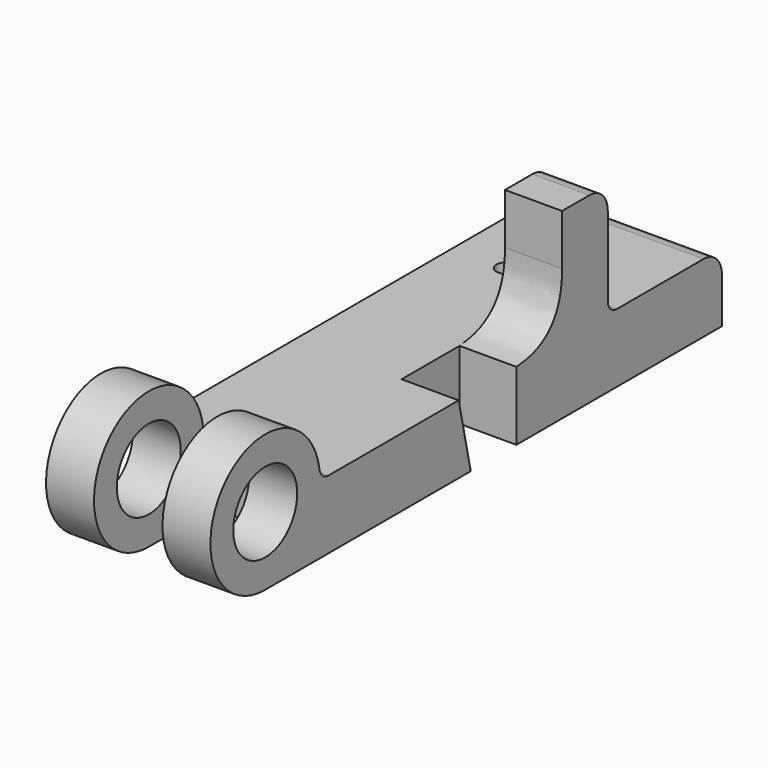
from build123d import *

# Parameters (mm, degrees)
F0_R         = 7
F1_DEPTH     = 14.4
F2_W         = 12
F2_H         = 26.4532811218
F2_H_2       = 2.4532811218
F3_DEPTH     = 15
F4_R         = 2
F6_DEPTH     = 25
F7_W         = 18.8
F7_H         = 33.2335345083
F7_H_2       = 13.5664814711
F8_DEPTH     = 25
F11_DEPTH    = 10
F12_T4_DEPTH = 10


# Not quite as in the source:
# - a fillet or chamfer that OpenCascade refuses, or shapes differently, is made with other operations: its cross-section is extruded or revolved along the edge and cut away or added


with BuildPart() as f1:
    # F0 (on Right) → F1 (new body, symmetric)
    with BuildSketch(Plane.YZ):
        with BuildLine():
            Line((42.36, 0), (12, 0))
            ThreePointArc((12, 0), (-8.4852813742, 8.4852813742), (0, -12))
            Line((0, -12), (47.36, -12))
            Line((47.36, -12), (42.36, 0))
        make_face()
        Circle(F0_R, mode=Mode.SUBTRACT)
        Polygon((57.36, 0), (42.36, 0), (47.36, -12), (57.36, -12), align=None)
        with BuildLine():
            Line((65, 0), (57.36, 0))
            Line((57.36, 0), (57.36, -12))
            Line((57.36, -12), (100, -12))
            Line((100, -12), (100, -4))
            ThreePointArc((100, -4), (98.8284271247, -1.1715728753), (96, 0))
            Line((96, 0), (77, 0))
            ThreePointArc((77, 0), (75.5857864376, 0.5857864376), (75, 2))
            Line((75, 2), (75, 16))
            ThreePointArc((75, 16), (73.8284271247, 18.8284271247), (71, 20))
            Line((71, 20), (65, 20))
            Line((65, 20), (65, 0))
        make_face()
    extrude(amount=F1_DEPTH, both=True)

    # F2 (on face) → F3 (cut, symmetric)
    with BuildSketch(Plane.XY):
        with Locations((0, -1.2266405609)):
            Rectangle(F2_W, F2_H)
        with Locations((0, 13.2266405609)):
            Rectangle(F2_W, F2_H_2)
    extrude(amount=F3_DEPTH, both=True, mode=Mode.SUBTRACT)

    # F4
    f4_edges = [f1.edges().sort_by_distance(p)[0] for p in [
        (10.2, 12, 0),
        (-10.2, 12, 0),
    ]]
    fillet(f4_edges, radius=F4_R)

    # F5 (on face) → F6 (cut)
    with BuildSketch(Plane.XY):
        with BuildLine():
            Line((-5, 77), (-6.7, 77))
            ThreePointArc((-6.7, 77), (-5, 75.3), (-3.3, 77))
            Line((-3.3, 77), (-5, 77))
        make_face()
        with BuildLine():
            ThreePointArc((-3.3, 77), (-5, 78.7), (-6.7, 77))
            Line((-6.7, 77), (-5, 77))
            Line((-5, 77), (-3.3, 77))
        make_face()
    extrude(amount=-F6_DEPTH, mode=Mode.SUBTRACT)

    # F7 (on face) → F8 (cut)
    with BuildSketch(Plane.XY):
        with Locations((-5, 81.6167672542)):
            Rectangle(F7_W, F7_H)
        with Locations((-5, 58.2167592645)):
            Rectangle(F7_W, F7_H_2)
    extrude(amount=F8_DEPTH, mode=Mode.SUBTRACT)

    # F10 (on face) → F11 (cut)
    with BuildSketch(Plane.YZ.offset(14.4)):
        Polygon((55, -12), (55, 0), (42.36, 0), (45, -12), align=None)
    extrude(amount=-F11_DEPTH, mode=Mode.SUBTRACT)

    # F12: fillet of radius 11.1053823869 on 1 edges, made by hand


with BuildPart() as f12_tool2:
    # F12_s3 → F12_t4 (new body)
    with BuildSketch(Plane.YZ.offset(14.4)):
        with BuildLine():
            add(Edge.make_bspline(
                [(53.8946176131, 0), (65, 0), (65, 11.1053823869)],
                knots=[0, 0, 0, 1, 1, 1], degree=2, weights=[1, 1, 1]))
            Line((65, 11.1053823869), (65, 0))
            Line((65, 0), (53.8946176131, 0))
        make_face()
    extrude(amount=-F12_T4_DEPTH)

    split(bisect_by=Plane.XZ.offset(-55), keep=Keep.BOTTOM)


with BuildPart() as f1_1:
    add(f1.part)

    # F12_t1: union F12_tool2
    add(f12_tool2.part)


solid = f1_1.part
